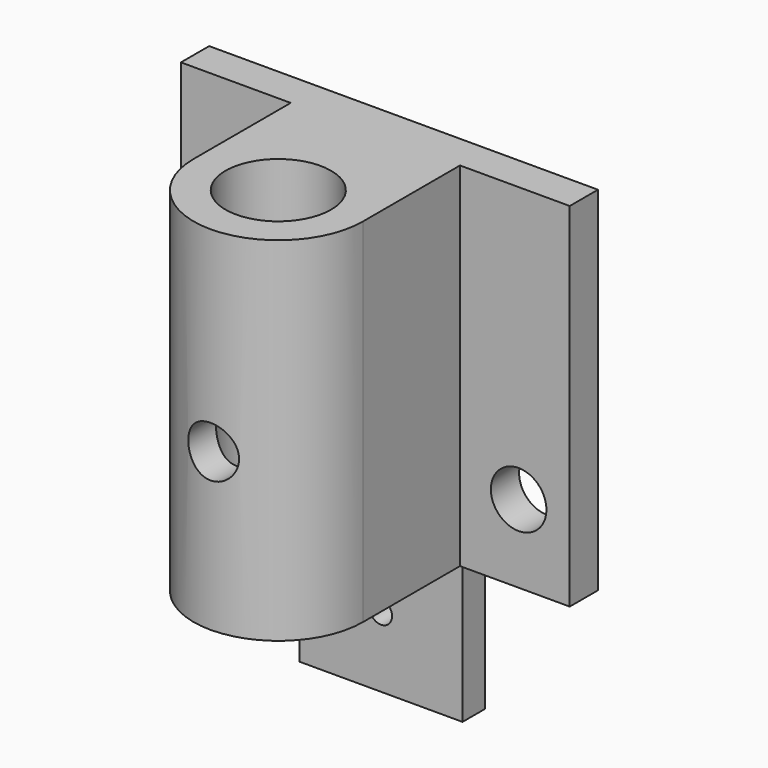
from build123d import *

# Parameters (mm, degrees)
F1_DEPTH = 31.75
F2_R     = 4.75
F3_DEPTH = 38.1
F5_D     = 4.572
F5_DEPTH = 7.621
F7_DEPTH = 12.7
F9_D     = 2
F11_D    = 5


# Not quite as in the source:
# - a feature names something its author has since deleted; it is built from what else it names


with BuildPart() as f1:
    # F0 (on Top) → F1 (new body)
    with BuildSketch(Plane.XY):
        with BuildLine():
            Line((-7.62, 10.9198254229), (-7.62, 0))
            ThreePointArc((-7.62, 0), (0, -7.62), (7.62, 0))
            Line((7.62, 0), (7.62, 10.9198254229))
            Line((7.62, 10.9198254229), (17.5, 10.9198254229))
            Line((17.5, 10.9198254229), (17.5, 14.0948254229))
            Line((17.5, 14.0948254229), (-17.5, 14.0948254229))
            Line((-17.5, 14.0948254229), (-17.5, 10.9198254229))
            Line((-17.5, 10.9198254229), (-7.62, 10.9198254229))
        make_face()
    extrude(amount=F1_DEPTH)

    # F2 (on face) → F3 (cut)
    with BuildSketch(Plane(origin=(0, 0, 0), x_dir=(1, 0, 0), z_dir=(0, 0, -1))):
        Circle(F2_R)
    extrude(amount=-F3_DEPTH, mode=Mode.SUBTRACT)

    # F5 (through all, one way)
    with BuildSketch(Plane(origin=(0, 0, 0), x_dir=(1, 0, 0), z_dir=(0, 1, 0))):
        with Locations((0, -14.1290773165)):
            Circle(F5_D / 2)
    extrude(amount=-F5_DEPTH, mode=Mode.SUBTRACT)

    # F6 (on face) → F7 (join)
    with BuildSketch(Plane(origin=(0, 0, 0), x_dir=(1, 0, 0), z_dir=(0, 0, -1))):
        Polygon((-7.34, -11.5548254229), (-7.34, -14.0948254229), (0, -14.0948254229), (7.34, -14.0948254229), (7.34, -11.5548254229), (0, -11.5548254229), align=None)
    extrude(amount=F7_DEPTH)

    # F9 (through all)
    with Locations(Plane.XZ.offset(-11.5548254229)):
        with Locations((0, -6.3856272027)):
            Hole(F9_D / 2)

    # F11 (through all)
    with Locations(Plane.XZ.offset(-10.9198254229)):
        with Locations((-12.9, 6.9917379814), (12.9, 6.9917379814)):
            Hole(F11_D / 2)


solid = f1.part
